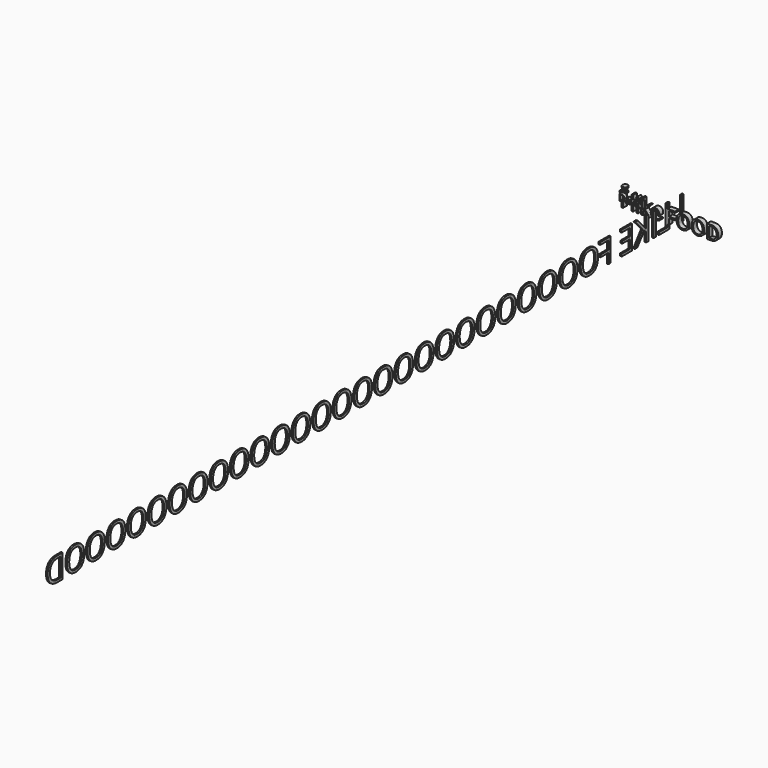
from build123d import *

# Parameters (mm, degrees)
F1_DEPTH      = 76.2
F2_R          = 23.7466929554
F3_DEPTH      = 63.501
F4_W          = 61.2166747451
F4_H          = 10.2439690381
F5_DEPTH      = 40.894
F6_R          = 43.2434785892
F7_DEPTH      = 18.542
F8_TEXT_SIZE  = 39.7913468381
F9_DEPTH      = 25.4
F10_TEXT_SIZE = 146.8716654927
F11_DEPTH     = 50.8
F12_TEXT_SIZE = 307.769395618
F13_DEPTH     = 76.2
F14_TEXT_SIZE = 528.314192262
F15_DEPTH     = 25.4


# Not quite as in the source:
# - Text() gives the source's letters only with a copy of the font that has no kerning and outlines rounded to 1/6400 em; it was checked with that copy


with BuildPart() as f1:
    # F0 (on Front) → F1 (new body)
    with BuildSketch(Plane.XZ):
        Polygon((-45.3785472333, -27.3050943582), (-45.3785472333, -52.7050943582), (43.5214527667, -52.7050943582), (43.5214527667, -27.3050943582), (18.1214527667, -27.3050943582), (18.1214527667, 36.1949056418), (43.5214527667, 36.1949056418), (43.5214527667, 61.5949056418), (-45.3785472333, 61.5949056418), (-45.3785472333, 36.1949056418), (-19.9785472333, 36.1949056418), (-19.9785472333, -27.3050943582), align=None)
    extrude(amount=F1_DEPTH)

    # F2 (on face) → F3 (cut, through all)
    with BuildSketch(Plane(origin=(-19.9785472333, 0, 0), x_dir=(0, -1, 0), z_dir=(-1, 0, 0))):
        with Locations((38.1, 4.4449056418)):
            Circle(F2_R)
    extrude(amount=-F3_DEPTH, mode=Mode.SUBTRACT)

    # F4 (on face) → F5 (join)
    with BuildSketch(Plane.XY.offset(61.5949056418)):
        with Locations((-0.6141532212, -16.7706003413)):
            Rectangle(F4_W, F4_H)
    extrude(amount=F5_DEPTH)

    # F6 (on face) → F7 (join)
    with BuildSketch(Plane.XY.offset(102.4889056418)):
        with Locations((-0.6141532212, -15.1294711977)):
            Circle(F6_R)
    extrude(amount=F7_DEPTH)

    # F8 (on face) → F9 (join)
    with BuildSketch(Plane.XZ.offset(21.8925848603)):
        with Locations((-27.7170017362, 68.2823956013)):
            Text('HI', F8_TEXT_SIZE, font='Open Sans', font_style=FontStyle.BOLD, text_align=(TextAlign.LEFT, TextAlign.BOTTOM))
    extrude(amount=F9_DEPTH)

    # F10 (on face) → F11 (join)
    with BuildSketch(Plane.XZ.offset(76.2)):
        with Locations((-17.1597078443, -48.2395514846)):
            Text('David', F10_TEXT_SIZE, font='Open Sans', text_align=(TextAlign.LEFT, TextAlign.BOTTOM))
    extrude(amount=F11_DEPTH)


with BuildPart() as f13:
    # F12 (on Front) → F13 (new body)
    with BuildSketch(Plane.XZ):
        with Locations((-42.7651777864, -162.3437851667)):
            Text('I like FOOD', F12_TEXT_SIZE, font='Open Sans', text_align=(TextAlign.LEFT, TextAlign.BOTTOM))
    extrude(amount=F13_DEPTH)

    # F14 (on face) → F15 (join)
    with BuildSketch(Plane(origin=(723.0997276218, 0, 0), x_dir=(0, -1, 0), z_dir=(-1, 0, 0))):
        with Locations((-303.0905723572, -246.3125735521)):
            Text('I LIKE FOOOOOOOOOOOOOOOOOOOOOOOOOOD', F14_TEXT_SIZE, font='Open Sans', text_align=(TextAlign.LEFT, TextAlign.BOTTOM))
    extrude(amount=F15_DEPTH)


solid = Compound([f1.part, f13.part])
